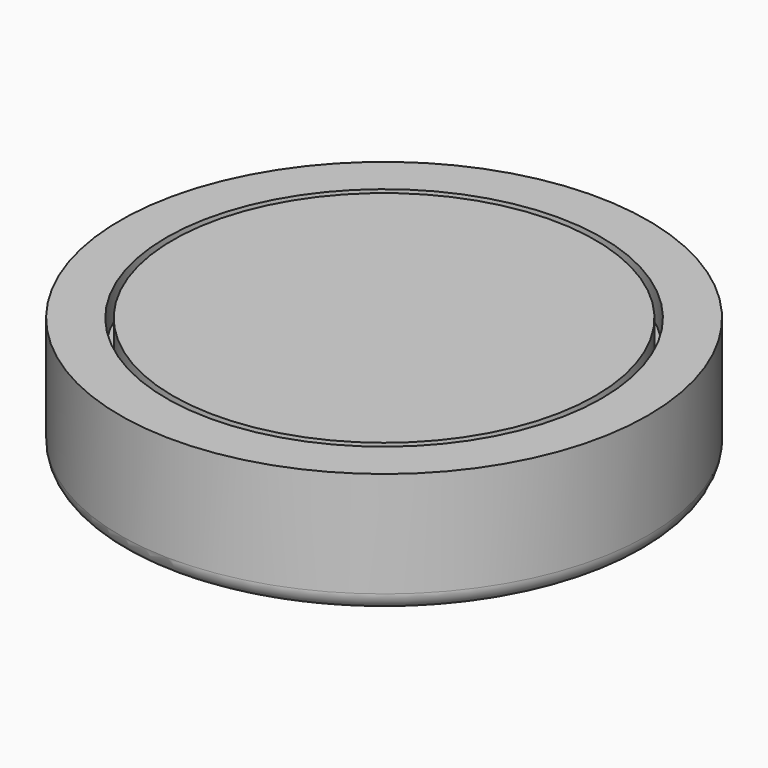
from build123d import *

# Parameters (mm, degrees)
F0_R      = 1.25
F1_DEPTH  = 3
F3_DEPTH  = 6
F4_R      = 1.2192
F5_DEPTH  = 7
F4_R_2    = 2
F4_R_3    = 0.9271
F7_R      = 24
F7_R_2    = 22
F7_R_3    = 21
F8_DEPTH  = 1.5
F9_DEPTH  = 2
F10_DEPTH = 2
F12_R     = 30
F12_R_2   = 24.75
F12_R_3   = 22.75
F12_R_4   = 2.75
F12_R_5   = 0.75
F12_R_6   = 1.875
F13_DEPTH = 2
F14_DEPTH = 1.5
F16_DEPTH = 8.5
F17_DEPTH = 12
F18_R     = 1.99999


# Not quite as in the source:
# - a fillet or chamfer that OpenCascade refuses, or shapes differently, is made with other operations: its cross-section is extruded or revolved along the edge and cut away or added
# - a fillet or chamfer is up to 0.001 mm smaller than in the source, because OpenCascade refuses the exact size


with BuildPart() as f1:
    # F0 (on Top) → F1 (new body)
    with BuildSketch(Plane.XY):
        with BuildLine():
            Line((8.25, 11.25), (8.25, 14.5))
            Line((8.25, 14.5), (-14.5, 14.5))
            Line((-14.5, 14.5), (-14.5, -8.25))
            Line((-14.5, -8.25), (-11.25, -8.25))
            ThreePointArc((-11.25, -8.25), (-9.1286796564, -9.1286796564), (-8.25, -11.25))
            Line((-8.25, -11.25), (-8.25, -14.5))
            Line((-8.25, -14.5), (14.5, -14.5))
            Line((14.5, -14.5), (14.5, 8.25))
            Line((14.5, 8.25), (11.25, 8.25))
            ThreePointArc((11.25, 8.25), (9.1286796564, 9.1286796564), (8.25, 11.25))
        make_face()
        with Locations((8.75, -11.75)):
            Circle(F0_R, mode=Mode.SUBTRACT)
        with Locations((-8.75, 11.75)):
            Circle(F0_R, mode=Mode.SUBTRACT)
    extrude(amount=-F1_DEPTH)

    # F2 (on Top) → F3 (join)
    with BuildSketch(Plane.XY):
        with BuildLine():
            ThreePointArc((7.5137790093, -9.675), (11.0024154817, -5.3860331941), (12.25, 0))
            ThreePointArc((12.25, 0), (11.0024154817, 5.3860331941), (7.5137790093, 9.675))
            Line((7.5137790093, 9.675), (-7.5137790093, 9.675))
            ThreePointArc((-7.5137790093, 9.675), (-12.25, 0), (-7.5137790093, -9.675))
            Line((-7.5137790093, -9.675), (7.5137790093, -9.675))
        make_face()
        with BuildLine():
            ThreePointArc((-7.5137790093, -9.675), (0, -12.25), (7.5137790093, -9.675))
            Line((7.5137790093, -9.675), (-7.5137790093, -9.675))
        make_face()
        with BuildLine():
            ThreePointArc((-7.5137790093, -9.675), (-12.25, 0), (-7.5137790093, 9.675))
            Line((-7.5137790093, 9.675), (-8.714591153, 9.675))
            Line((-8.714591153, 9.675), (-12.8, 7.175))
            Line((-12.8, 7.175), (-12.8, -5.5770184845))
            Line((-12.8, -5.5770184845), (-8.2916002721, -9.675))
            Line((-8.2916002721, -9.675), (-7.5137790093, -9.675))
        make_face()
        with BuildLine():
            ThreePointArc((7.5137790093, 9.675), (11.0024154817, 5.3860331941), (12.25, 0))
            ThreePointArc((12.25, 0), (11.0024154817, -5.3860331941), (7.5137790093, -9.675))
            Line((7.5137790093, -9.675), (7.8, -9.675))
            Line((7.8, -9.675), (12.8, -6.175))
            Line((12.8, -6.175), (12.8, 7.175))
            Line((12.8, 7.175), (8.17, 9.675))
            Line((8.17, 9.675), (7.5137790093, 9.675))
        make_face()
        with BuildLine():
            Line((-7.5137790093, 9.675), (7.5137790093, 9.675))
            ThreePointArc((7.5137790093, 9.675), (0, 12.25), (-7.5137790093, 9.675))
        make_face()
    extrude(amount=F3_DEPTH)


with BuildPart() as f5:
    # F4 (on Top) → F5 (new body)
    with BuildSketch(Plane.XY):
        with BuildLine():
            ThreePointArc((-9.1239573499, -12.75), (-8.9863719636, -12.2583896898), (-8.94, -11.75))
            ThreePointArc((-8.94, -11.75), (-8.9863719636, -11.2416103102), (-9.1239573499, -10.75))
            ThreePointArc((-9.1239573499, -10.75), (-9.7630299449, -9.7630299449), (-10.75, -9.1239573499))
            ThreePointArc((-10.75, -9.1239573499), (-11.75, -8.94), (-12.75, -9.1239573499))
            ThreePointArc((-12.75, -9.1239573499), (-13.7369700551, -13.7369700551), (-9.1239573499, -12.75))
        make_face()
        with Locations((-11.75, -11.75)):
            Circle(F4_R, mode=Mode.SUBTRACT)
        with BuildLine():
            ThreePointArc((-9.1239573499, -10.75), (-8.9863719636, -11.2416103102), (-8.94, -11.75))
            ThreePointArc((-8.94, -11.75), (-8.9863719636, -12.2583896898), (-9.1239573499, -12.75))
            Line((-9.1239573499, -12.75), (-8.75, -12.75))
            ThreePointArc((-8.75, -12.75), (-8.0428932188, -12.4571067812), (-7.75, -11.75))
            ThreePointArc((-7.75, -11.75), (-8.0428932188, -11.0428932188), (-8.75, -10.75))
            Line((-8.75, -10.75), (-9.1239573499, -10.75))
        make_face()
        with BuildLine():
            ThreePointArc((-12.75, -9.1239573499), (-11.75, -8.94), (-10.75, -9.1239573499))
            Line((-10.75, -9.1239573499), (-10.75, -8.75))
            ThreePointArc((-10.75, -8.75), (-11.0428932188, -8.0428932188), (-11.75, -7.75))
            ThreePointArc((-11.75, -7.75), (-12.4571067812, -8.0428932188), (-12.75, -8.75))
            Line((-12.75, -8.75), (-12.75, -9.1239573499))
        make_face()
    extrude(amount=F5_DEPTH)



with BuildPart() as f5b:
    # F4 (on Top) → F5, piece 2 (new body)
    with BuildSketch(Plane.XY):
        with Locations((8.75, -11.75)):
            Circle(F4_R_2)
        with Locations((8.75, -11.75)):
            Circle(F4_R_3, mode=Mode.SUBTRACT)
    extrude(amount=F5_DEPTH)


with BuildPart() as f5c:
    # F4 (on Top) → F5, piece 3 (new body)
    with BuildSketch(Plane.XY):
        with BuildLine():
            ThreePointArc((9.1239573499, 10.75), (8.94, 11.75), (9.1239573499, 12.75))
            Line((9.1239573499, 12.75), (8.75, 12.75))
            ThreePointArc((8.75, 12.75), (8.0428932188, 12.4571067812), (7.75, 11.75))
            ThreePointArc((7.75, 11.75), (8.0428932188, 11.0428932188), (8.75, 10.75))
            Line((8.75, 10.75), (9.1239573499, 10.75))
        make_face()
        with BuildLine():
            Line((12.75, 8.75), (12.75, 9.1239573499))
            ThreePointArc((12.75, 9.1239573499), (11.75, 8.94), (10.75, 9.1239573499))
            Line((10.75, 9.1239573499), (10.75, 8.75))
            ThreePointArc((10.75, 8.75), (11.0428932188, 8.0428932188), (11.75, 7.75))
            ThreePointArc((11.75, 7.75), (12.4571067812, 8.0428932188), (12.75, 8.75))
        make_face()
        with BuildLine():
            ThreePointArc((12.75, 9.1239573499), (14.0636659223, 10.1553056719), (14.56, 11.75))
            ThreePointArc((14.56, 11.75), (12.2583896898, 14.5136280364), (9.1239573499, 12.75))
            ThreePointArc((9.1239573499, 12.75), (8.94, 11.75), (9.1239573499, 10.75))
            ThreePointArc((9.1239573499, 10.75), (9.7630299449, 9.7630299449), (10.75, 9.1239573499))
            ThreePointArc((10.75, 9.1239573499), (11.75, 8.94), (12.75, 9.1239573499))
        make_face()
        with Locations((11.75, 11.75)):
            Circle(F4_R, mode=Mode.SUBTRACT)
    extrude(amount=F5_DEPTH)


with BuildPart() as f5d:
    # F4 (on Top) → F5, piece 4 (new body)
    with BuildSketch(Plane.XY):
        with Locations((-8.75, 11.75)):
            Circle(F4_R_2)
        with Locations((-8.75, 11.75)):
            Circle(F4_R_3, mode=Mode.SUBTRACT)
    extrude(amount=F5_DEPTH)


with BuildPart() as f5_1:
    add(f5.part)

    add(f5b.part)  # F8 merges F5b

    add(f5c.part)  # F8 merges F5c

    add(f5d.part)  # F8 merges F5d
    # F7 (on offset) → F8 (join)
    with BuildSketch(Plane.XY.offset(7)):
        Circle(F7_R)
        Circle(F7_R_2, mode=Mode.SUBTRACT)
        Circle(F7_R_2)
        Circle(F7_R_3, mode=Mode.SUBTRACT)
        Circle(F7_R_3)
    extrude(amount=F8_DEPTH)

    # F4 (on Top) → F9 (join)
    with BuildSketch(Plane.XY):
        with BuildLine():
            ThreePointArc((-9.1239573499, -12.75), (-8.9863719636, -12.2583896898), (-8.94, -11.75))
            ThreePointArc((-8.94, -11.75), (-8.9863719636, -11.2416103102), (-9.1239573499, -10.75))
            ThreePointArc((-9.1239573499, -10.75), (-9.7630299449, -9.7630299449), (-10.75, -9.1239573499))
            ThreePointArc((-10.75, -9.1239573499), (-11.75, -8.94), (-12.75, -9.1239573499))
            ThreePointArc((-12.75, -9.1239573499), (-13.7369700551, -13.7369700551), (-9.1239573499, -12.75))
        make_face()
        with Locations((-11.75, -11.75)):
            Circle(F4_R, mode=Mode.SUBTRACT)
        with BuildLine():
            ThreePointArc((12.75, 9.1239573499), (14.0636659223, 10.1553056719), (14.56, 11.75))
            ThreePointArc((14.56, 11.75), (12.2583896898, 14.5136280364), (9.1239573499, 12.75))
            ThreePointArc((9.1239573499, 12.75), (8.94, 11.75), (9.1239573499, 10.75))
            ThreePointArc((9.1239573499, 10.75), (9.7630299449, 9.7630299449), (10.75, 9.1239573499))
            ThreePointArc((10.75, 9.1239573499), (11.75, 8.94), (12.75, 9.1239573499))
        make_face()
        with Locations((11.75, 11.75)):
            Circle(F4_R, mode=Mode.SUBTRACT)
    extrude(amount=-F9_DEPTH)

    # F7 (on offset) → F10 (join)
    with BuildSketch(Plane.XY.offset(7)):
        Circle(F7_R)
        Circle(F7_R_2, mode=Mode.SUBTRACT)
    extrude(amount=-F10_DEPTH)


with BuildPart() as f13:
    # F12 (on offset) → F13 (new body)
    with BuildSketch(Plane(origin=(0, 0, -3.5), x_dir=(1, 0, 0), z_dir=(0, 0, -1))):
        Circle(F12_R)
        Circle(F12_R_2, mode=Mode.SUBTRACT)
        Circle(F12_R_2)
        Circle(F12_R_3, mode=Mode.SUBTRACT)
        Circle(F12_R_3)
        with Locations((11.75, -11.75)):
            Circle(F12_R_4, mode=Mode.SUBTRACT)
        with Locations((-11.75, 11.75)):
            Circle(F12_R_4, mode=Mode.SUBTRACT)
        with Locations((1.5, 1.5)):
            Circle(F12_R_5, mode=Mode.SUBTRACT)
        with Locations((-11.75, 11.75)):
            Circle(F12_R_4)
        with Locations((-11.75, 11.75)):
            Circle(F12_R_6, mode=Mode.SUBTRACT)
        with Locations((11.75, -11.75)):
            Circle(F12_R_4)
        with Locations((11.75, -11.75)):
            Circle(F12_R_6, mode=Mode.SUBTRACT)
    extrude(amount=F13_DEPTH)

    # F12 (on offset) → F14 (join)
    with BuildSketch(Plane(origin=(0, 0, -3.5), x_dir=(1, 0, 0), z_dir=(0, 0, -1))):
        with Locations((11.75, -11.75)):
            Circle(F12_R_4)
        with Locations((11.75, -11.75)):
            Circle(F12_R_6, mode=Mode.SUBTRACT)
        with Locations((-11.75, 11.75)):
            Circle(F12_R_4)
        with Locations((-11.75, 11.75)):
            Circle(F12_R_6, mode=Mode.SUBTRACT)
    extrude(amount=-F14_DEPTH)

    # F15: chamfer of 2 on 2 edges, made by hand

    # F15_s1 → F15_t2 (revolve, cut)
    with BuildSketch(Plane.XZ.offset(11.75)):
        Polygon((-7.875, -5.5), (-9.875, -3.5), (-9.875, -5.5), align=None)
    revolve(axis=Axis((-11.75, -11.75, -5.5), (0, 0, -1)), mode=Mode.SUBTRACT)

    # F15_s3 → F15_t4 (revolve, cut)
    with BuildSketch(Plane.XZ.offset(-11.75)):
        Polygon((15.625, -5.5), (13.625, -3.5), (13.625, -5.5), align=None)
    revolve(axis=Axis((11.75, 11.75, -5.5), (0, 0, -1)), mode=Mode.SUBTRACT)

    # F12 (on offset) → F16 (join, through all)
    with BuildSketch(Plane(origin=(0, 0, -3.5), x_dir=(1, 0, 0), z_dir=(0, 0, -1))):
        Circle(F12_R_2)
        Circle(F12_R_3, mode=Mode.SUBTRACT)
    extrude(amount=-F16_DEPTH)

    # F12 (on offset) → F17 (join)
    with BuildSketch(Plane(origin=(0, 0, -3.5), x_dir=(1, 0, 0), z_dir=(0, 0, -1))):
        Circle(F12_R)
        Circle(F12_R_2, mode=Mode.SUBTRACT)
    extrude(amount=-F17_DEPTH)

    # F18 (radius 2 in the source; OpenCascade refuses exactly that, so slightly less here)
    f18_edges = [f13.edges().sort_by_distance(p)[0] for p in [
        (-30, 0, -5.5),
    ]]
    fillet(f18_edges, radius=F18_R)


solid = Compound([f1.part, f5_1.part, f13.part])
